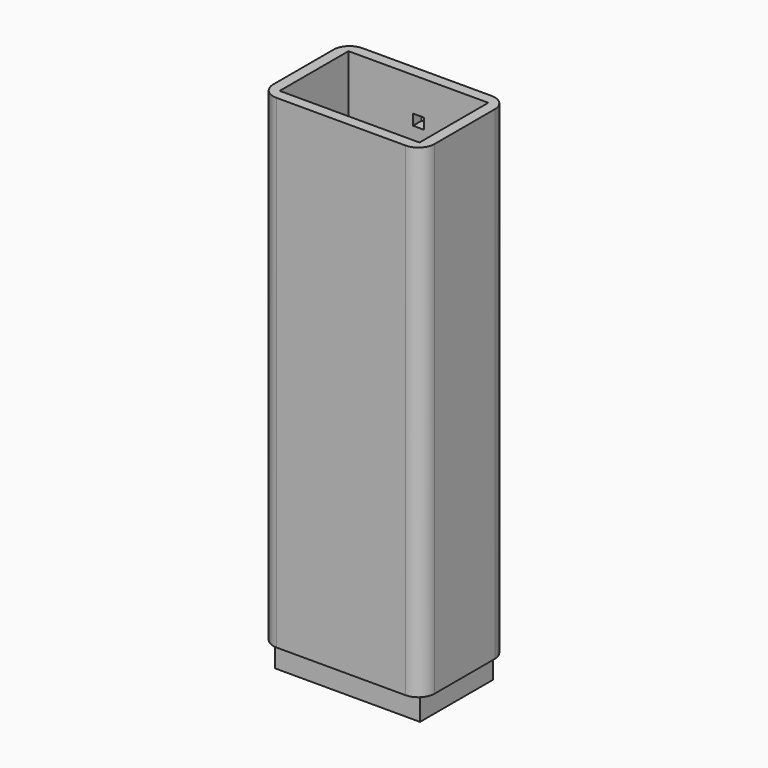
from build123d import *

# Parameters (mm, degrees)
F0_W      = 30
F0_H      = 20
F1_DEPTH  = 90
F2_R      = 3
F3_W      = 26
F3_H      = 16
F4_DEPTH  = 100
F5_W      = 27
F5_H      = 17
F6_DEPTH  = 4.5
F7_DEPTH  = 5
F8_R      = 3.0778907451
F8_W      = 2
F8_H      = 2
F9_DEPTH  = 2
F10_W     = 7
F10_H     = 7
F11_DEPTH = 0.5
F12_W     = 26
F12_H     = 8.5281978436
F13_DEPTH = 2
F14_W     = 14
F14_H     = 8.5281978436
F15_DEPTH = 2
F16_W     = 24
F16_H     = 8.5281978436
F17_DEPTH = 2
F18_W     = 12
F18_H     = 8.5281978436
F19_DEPTH = 2
F20_R     = 1.99999


# Not quite as in the source:
# - a fillet or chamfer is up to 0.001 mm smaller than in the source, because OpenCascade refuses the exact size


with BuildPart() as f1:
    # F0 (on Top) → F1 (new body)
    with BuildSketch(Plane.XY):
        with Locations((-4.6270154417, 7.9813233296)):
            Rectangle(F0_W, F0_H)
    extrude(amount=F1_DEPTH)

    # F2
    f2_edges = [f1.edges().sort_by_distance(p)[0] for p in [
        (-19.627015, -2.018677, 45),
        (-19.627015, 17.981323, 45),
        (10.372985, -2.018677, 45),
        (10.372985, 17.981323, 45),
    ]]
    fillet(f2_edges, radius=F2_R)

    # F3 (on face) → F4 (cut)
    with BuildSketch(Plane.XY.offset(90)):
        with Locations((-4.6270154417, 7.9813233296)):
            Rectangle(F3_W, F3_H)
    extrude(amount=-F4_DEPTH, mode=Mode.SUBTRACT)

    # F5 (on face) → F6 (join)
    with BuildSketch(Plane(origin=(0, 0, 0), x_dir=(1, 0, 0), z_dir=(0, 0, -1))):
        with Locations((-4.6270154417, -7.9813233296)):
            Rectangle(F5_W, F5_H)
    extrude(amount=F6_DEPTH)

    # F7 (cut): a face of the model
    f7_faces = [f1.faces().sort_by_distance(p)[0] for p in [
        (-4.6270154417, 7.9813233296, 0),
    ]]
    extrude(f7_faces, amount=-F7_DEPTH, mode=Mode.SUBTRACT)

    # F8 (on face) → F9 (cut)
    with BuildSketch(Plane(origin=(0, 17.9813233296, 0), x_dir=(-1, 0, 0), z_dir=(0, 1, 0))):
        with Locations((4.6270154417, 71.1657330394)):
            Circle(F8_R)
        with Locations((4.6270154417, 82.6890671849)):
            Rectangle(F8_W, F8_H)
    extrude(amount=-F9_DEPTH, mode=Mode.SUBTRACT)

    # F10 (on face) → F11 (cut)
    with BuildSketch(Plane.XZ.offset(-15.9813233296)):
        with Locations((-4.6607098193, 71.1224186855)):
            Rectangle(F10_W, F10_H)
    extrude(amount=-F11_DEPTH, mode=Mode.SUBTRACT)

    # F12 (on face) → F13 (join)
    with BuildSketch(Plane.XZ.offset(-15.9813233296)):
        with Locations((-4.6270154417, -0.2359010782)):
            Rectangle(F12_W, F12_H)
    extrude(amount=F13_DEPTH)

    # F14 (on face) → F15 (join)
    with BuildSketch(Plane(origin=(8.3729845583, 0, 0), x_dir=(0, -1, 0), z_dir=(-1, 0, 0))):
        with Locations((-6.9813233296, -0.2359010782)):
            Rectangle(F14_W, F14_H)
    extrude(amount=F15_DEPTH)

    # F16 (on face) → F17 (join)
    with BuildSketch(Plane(origin=(0, -0.0186766704, 0), x_dir=(-1, 0, 0), z_dir=(0, 1, 0))):
        with Locations((5.6270154417, -0.2359010782)):
            Rectangle(F16_W, F16_H)
    extrude(amount=F17_DEPTH)

    # F18 (on face) → F19 (join)
    with BuildSketch(Plane.YZ.offset(-17.6270154417)):
        with Locations((7.9813233296, -0.2359010782)):
            Rectangle(F18_W, F18_H)
    extrude(amount=F19_DEPTH)

    # F20 (radius 2 in the source; OpenCascade refuses exactly that, so slightly less here)
    f20_edges = [f1.edges().sort_by_distance(p)[0] for p in [
        (-15.627015, 7.981323, 4.028198),
        (-4.627015, 1.981323, 4.028198),
        (6.372985, 7.981323, 4.028198),
        (-4.627015, 13.981323, 4.028198),
    ]]
    fillet(f20_edges, radius=F20_R)


solid = f1.part
